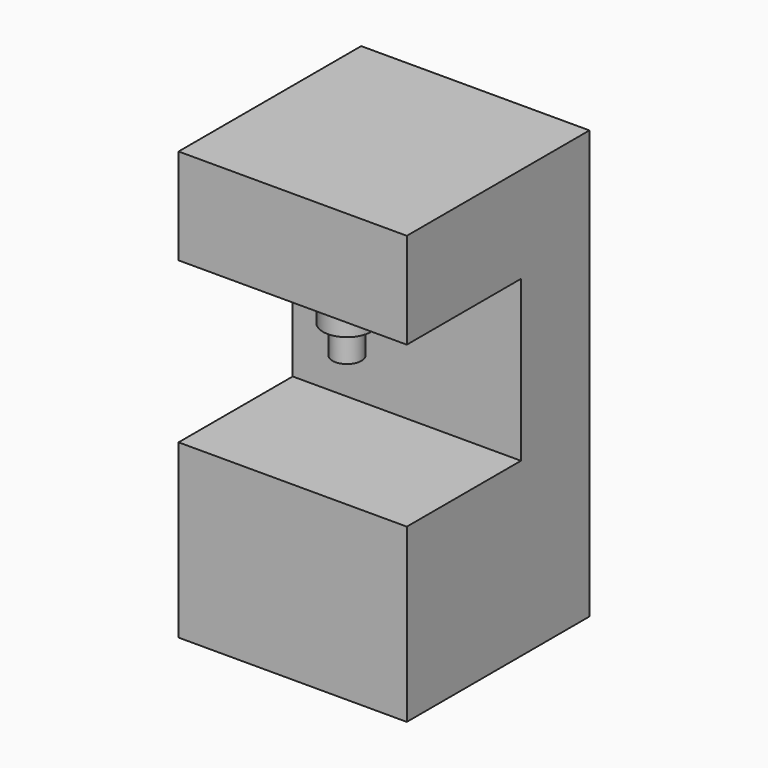
from build123d import *

# Parameters (mm, degrees)
F0_W     = 1016
F0_H     = 1905
F1_DEPTH = 1016
F2_W     = 1016
F2_H     = 713.0777835846
F3_DEPTH = 635
F4_R     = 106.5109159408
F5_DEPTH = 193.04
F6_R     = 64.5918203827
F7_DEPTH = 127


# Not quite as in the source:
# - the program builds the solid bodies; features that only make, move or delete a surface that nothing else refers to are left out


with BuildPart() as f1:
    # F0 (on Front) → F1 (new body)
    with BuildSketch(Plane.XZ):
        with Locations((-508, 952.5)):
            Rectangle(F0_W, F0_H)
    extrude(amount=F1_DEPTH)

    # F2 (on face) → F3 (cut)
    with BuildSketch(Plane.XZ.offset(1016)):
        with Locations((-508, 1121.7548847198)):
            Rectangle(F2_W, F2_H)
    extrude(amount=-F3_DEPTH, mode=Mode.SUBTRACT)

    # F4 (on face) → F5 (join)
    with BuildSketch(Plane(origin=(0, 0, 1478.2937765121), x_dir=(1, 0, 0), z_dir=(0, 0, -1))):
        with Locations((-495.6358075142, 729.4123768806)):
            Circle(F4_R)
    extrude(amount=F5_DEPTH)

    # F6 (on face) → F7 (join)
    with BuildSketch(Plane(origin=(0, 0, 1285.2537765121), x_dir=(1, 0, 0), z_dir=(0, 0, -1))):
        with Locations((-495.6358075142, 729.4123768806)):
            Circle(F6_R)
    extrude(amount=F7_DEPTH)


solid = f1.part
